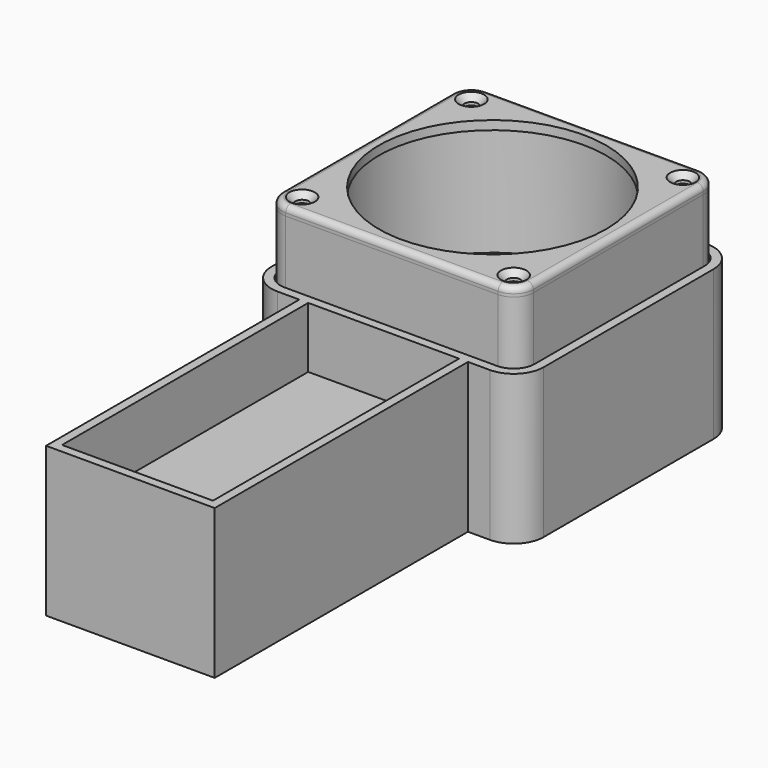
from build123d import *

# Parameters (mm, degrees)
F0_W      = 80
F0_H      = 80
F0_R      = 2.1
F0_R_2    = 38.4
F1_DEPTH  = 25
F2_W      = 79.6
F2_H      = 79.6
F2_R      = 2.3
F2_R_2    = 38.6
F3_DEPTH  = 1.5875
F4_W      = 79.6
F4_H      = 79.6
F4_R      = 2.3
F4_R_2    = 38.6
F5_DEPTH  = 1.5875
F8_W      = 92
F8_H      = 92
F8_W_2    = 86
F8_H_2    = 86
F9_DEPTH  = 27.54
F10_W     = 92
F10_H     = 92
F10_R     = 2.3
F10_R_2   = 38.4
F11_DEPTH = 3
F12_SIZE  = 2
F13_W     = 92
F13_H     = 92
F13_W_2   = 86
F13_H_2   = 86
F14_DEPTH = 20
F15_R     = 42.4
F15_R_2   = 38.4
F16_DEPTH = 1.27
F17_R     = 42.2
F17_R_2   = 38.6
F18_DEPTH = 1.5875
F19_W     = 85
F19_H     = 85
F19_R     = 38.4
F20_DEPTH = 41
F21_R     = 41.4
F22_DEPTH = 38
F23_R     = 3.25
F24_DEPTH = 12.7
F25_R     = 3.15
F26_DEPTH = 6.7
F27_R     = 3.6661742094
F28_DEPTH = 0.5
F30_DEPTH = 71.8585
F31_R     = 6.6
F32_R     = 2
F33_R     = 2.3
F33_R_2   = 38.4
F34_DEPTH = 3
F35_SIZE  = 2
F36_R     = 2
F37_R     = 7.1
F38_R     = 10.1
F39_R     = 7.1
F40_W     = 57
F40_H     = 107
F41_DEPTH = 30
F42_W     = 51
F42_H     = 104
F43_DEPTH = 27
F44_W     = 57
F44_H     = 110
F44_W_2   = 51
F44_H_2   = 104
F45_DEPTH = 20.54


with BuildPart() as f1:
    # F0 (on Top) → F1 (new body)
    with BuildSketch(Plane.XY):
        Rectangle(F0_W, F0_H)
        with Locations((-35.75, -35.75)):
            Circle(F0_R, mode=Mode.SUBTRACT)
        with Locations((35.75, -35.75)):
            Circle(F0_R, mode=Mode.SUBTRACT)
        with Locations((-35.75, 35.75)):
            Circle(F0_R, mode=Mode.SUBTRACT)
        Circle(F0_R_2, mode=Mode.SUBTRACT)
        with Locations((35.75, 35.75)):
            Circle(F0_R, mode=Mode.SUBTRACT)
    extrude(amount=F1_DEPTH)


with BuildPart() as f3:
    # F2 (on face) → F3 (new body)
    with BuildSketch(Plane.XY.offset(25)):
        Rectangle(F2_W, F2_H)
        with Locations((-35.75, -35.75)):
            Circle(F2_R, mode=Mode.SUBTRACT)
        with Locations((35.75, -35.75)):
            Circle(F2_R, mode=Mode.SUBTRACT)
        with Locations((-35.75, 35.75)):
            Circle(F2_R, mode=Mode.SUBTRACT)
        Circle(F2_R_2, mode=Mode.SUBTRACT)
        with Locations((35.75, 35.75)):
            Circle(F2_R, mode=Mode.SUBTRACT)
    extrude(amount=F3_DEPTH)


with BuildPart() as f5:
    # F4 (on face) → F5 (new body)
    with BuildSketch(Plane(origin=(0, 0, 0), x_dir=(1, 0, 0), z_dir=(0, 0, -1))):
        Rectangle(F4_W, F4_H)
        with Locations((-35.75, -35.75)):
            Circle(F4_R, mode=Mode.SUBTRACT)
        with Locations((35.75, -35.75)):
            Circle(F4_R, mode=Mode.SUBTRACT)
        with Locations((-35.75, 35.75)):
            Circle(F4_R, mode=Mode.SUBTRACT)
        Circle(F4_R_2, mode=Mode.SUBTRACT)
        with Locations((35.75, 35.75)):
            Circle(F4_R, mode=Mode.SUBTRACT)
    extrude(amount=F5_DEPTH)


with BuildPart() as f9:
    # F8 (on offset) → F9 (new body, through all)
    with BuildSketch(Plane.XY.offset(26.27)):
        Rectangle(F8_W, F8_H)
        Rectangle(F8_W_2, F8_H_2, mode=Mode.SUBTRACT)
    extrude(amount=-F9_DEPTH)

    # F10 (on face) → F11 (join)
    with BuildSketch(Plane.XY.offset(26.27)):
        Rectangle(F10_W, F10_H)
        with Locations((-35.75, -35.75)):
            Circle(F10_R, mode=Mode.SUBTRACT)
        with Locations((35.75, -35.75)):
            Circle(F10_R, mode=Mode.SUBTRACT)
        with Locations((-35.75, 35.75)):
            Circle(F10_R, mode=Mode.SUBTRACT)
        Circle(F10_R_2, mode=Mode.SUBTRACT)
        with Locations((35.75, 35.75)):
            Circle(F10_R, mode=Mode.SUBTRACT)
    extrude(amount=F11_DEPTH)

    # F12
    f12_edges = [f9.edges().sort_by_distance(p)[0] for p in [
        (33.45, 35.75, 29.27),
        (33.45, -35.75, 29.27),
        (-38.05, -35.75, 29.27),
        (-38.05, 35.75, 29.27),
    ]]
    chamfer(f12_edges, length=F12_SIZE)

    # F13 (on face) → F14 (join)
    with BuildSketch(Plane.XY.offset(29.27)):
        Rectangle(F13_W, F13_H)
        Rectangle(F13_W_2, F13_H_2, mode=Mode.SUBTRACT)
    extrude(amount=F14_DEPTH)

    # F15 (on face) → F16 (cut)
    with BuildSketch(Plane.XY.offset(29.27)):
        Circle(F15_R)
        Circle(F15_R_2, mode=Mode.SUBTRACT)
    extrude(amount=-F16_DEPTH, mode=Mode.SUBTRACT)

    # F37
    f37_edges = [f9.edges().sort_by_distance(p)[0] for p in [
        (-43, -43, 39.27),
        (-43, 43, 39.27),
        (43, 43, 39.27),
        (43, -43, 39.27),
    ]]
    fillet(f37_edges, radius=F37_R)

    # F38
    f38_edges = [f9.edges().sort_by_distance(p)[0] for p in [
        (46, -46, 24),
        (46, 46, 24),
        (-46, 46, 24),
        (-46, -46, 24),
    ]]
    fillet(f38_edges, radius=F38_R)

    # F39
    f39_edges = [f9.edges().sort_by_distance(p)[0] for p in [
        (-43, -43, 12.5),
        (43, -43, 12.5),
        (-43, 43, 12.5),
        (43, 43, 12.5),
    ]]
    fillet(f39_edges, radius=F39_R)

    # F40 (on face) → F41 (join)
    with BuildSketch(Plane(origin=(0, 0, -1.27), x_dir=(1, 0, 0), z_dir=(0, 0, -1))):
        with Locations((0, 99.5)):
            Rectangle(F40_W, F40_H)
    extrude(amount=-F41_DEPTH)

    # F42 (on face) → F43 (cut)
    with BuildSketch(Plane(origin=(0, 0, -1.27), x_dir=(1, 0, 0), z_dir=(0, 0, -1))):
        with Locations((0, 98)):
            Rectangle(F42_W, F42_H)
    extrude(amount=-F43_DEPTH, mode=Mode.SUBTRACT)

    # F44 (on face) → F45 (join, through all)
    with BuildSketch(Plane.XY.offset(28.73)):
        with Locations((0, -98)):
            Rectangle(F44_W, F44_H)
        with Locations((0, -98)):
            Rectangle(F44_W_2, F44_H_2, mode=Mode.SUBTRACT)
    extrude(amount=F45_DEPTH)


with BuildPart() as f18:
    # F17 (on face) → F18 (new body)
    with BuildSketch(Plane.XY.offset(28)):
        Circle(F17_R)
        Circle(F17_R_2, mode=Mode.SUBTRACT)
    extrude(amount=F18_DEPTH)


with BuildPart() as f20:
    # F19 (on face) → F20 (new body)
    with BuildSketch(Plane.XY.offset(29.27)):
        Rectangle(F19_W, F19_H)
        Circle(F19_R, mode=Mode.SUBTRACT)
    extrude(amount=F20_DEPTH)

    # F21 (on face) → F22 (cut)
    with BuildSketch(Plane.XY.offset(70.27)):
        Circle(F21_R)
    extrude(amount=-F22_DEPTH, mode=Mode.SUBTRACT)

    # F23 (on face) → F24 (cut)
    with BuildSketch(Plane(origin=(0, 0, 29.27), x_dir=(1, 0, 0), z_dir=(0, 0, -1))):
        with Locations((35.75, -35.75)):
            Circle(F23_R)
        with Locations((-35.75, 35.75)):
            Circle(F23_R)
        with Locations((-35.75, -35.75)):
            Circle(F23_R)
        with Locations((35.75, 35.75)):
            Circle(F23_R)
    extrude(amount=-F24_DEPTH, mode=Mode.SUBTRACT)

    # F25 (on face) → F26 (cut)
    with BuildSketch(Plane.XY.offset(70.27)):
        with Locations((-35.75, 35.75)):
            Circle(F25_R)
        with Locations((35.75, 35.75)):
            Circle(F25_R)
        with Locations((35.75, -35.75)):
            Circle(F25_R)
        with Locations((-35.75, -35.75)):
            Circle(F25_R)
    extrude(amount=-F26_DEPTH, mode=Mode.SUBTRACT)

    # F27 (on face) → F28 (cut)
    with BuildSketch(Plane.XY.offset(70.27)):
        with Locations((-35.75, 35.75)):
            Circle(F27_R)
        with Locations((-35.75, -35.75)):
            Circle(F27_R)
        with Locations((35.75, -35.75)):
            Circle(F27_R)
        with Locations((35.75, 35.75)):
            Circle(F27_R)
    extrude(amount=-F28_DEPTH, mode=Mode.SUBTRACT)

    # F29 (on face) → F30 (cut, through all)
    with BuildSketch(Plane.XY.offset(70.27)):
        with BuildLine():
            ThreePointArc((-33.040767305, 29.659192435), (-36.3455933225, 29.1104859226), (-39.5, 30.2386137325))
            Line((-39.5, 30.2386137325), (-39.5, 20.2758477011))
            ThreePointArc((-39.5, 20.2758477011), (-36.572565126, 25.1755333628), (-33.040767305, 29.659192435))
        make_face()
        with BuildLine():
            ThreePointArc((-33.040767305, -29.659192435), (-36.572565126, -25.1755333628), (-39.5, -20.2758477011))
            Line((-39.5, -20.2758477011), (-39.5, -30.2386137325))
            ThreePointArc((-39.5, -30.2386137325), (-36.3455933225, -29.1104859226), (-33.040767305, -29.659192435))
        make_face()
        with BuildLine():
            ThreePointArc((-30.2386137325, 39.5), (-29.1104859226, 36.3455933225), (-29.659192435, 33.040767305))
            ThreePointArc((-29.659192435, 33.040767305), (-25.1755333628, 36.572565126), (-20.2758477011, 39.5))
            Line((-20.2758477011, 39.5), (-30.2386137325, 39.5))
        make_face()
        with BuildLine():
            ThreePointArc((-29.659192435, -33.040767305), (-29.1104859226, -36.3455933225), (-30.2386137325, -39.5))
            Line((-30.2386137325, -39.5), (-20.2758477011, -39.5))
            ThreePointArc((-20.2758477011, -39.5), (-25.1755333628, -36.572565126), (-29.659192435, -33.040767305))
        make_face()
        with BuildLine():
            ThreePointArc((29.659192435, -33.040767305), (25.1755333628, -36.572565126), (20.2758477011, -39.5))
            Line((20.2758477011, -39.5), (30.2386137325, -39.5))
            ThreePointArc((30.2386137325, -39.5), (29.1104859226, -36.3455933225), (29.659192435, -33.040767305))
        make_face()
        with BuildLine():
            ThreePointArc((33.040767305, -29.659192435), (36.3455933225, -29.1104859226), (39.5, -30.2386137325))
            Line((39.5, -30.2386137325), (39.5, -20.2758477011))
            ThreePointArc((39.5, -20.2758477011), (36.572565126, -25.1755333628), (33.040767305, -29.659192435))
        make_face()
        with BuildLine():
            ThreePointArc((33.040767305, 29.659192435), (36.572565126, 25.1755333628), (39.5, 20.2758477011))
            Line((39.5, 20.2758477011), (39.5, 30.2386137325))
            ThreePointArc((39.5, 30.2386137325), (36.3455933225, 29.1104859226), (33.040767305, 29.659192435))
        make_face()
        with BuildLine():
            ThreePointArc((29.659192435, 33.040767305), (29.1104859226, 36.3455933225), (30.2386137325, 39.5))
            Line((30.2386137325, 39.5), (20.2758477011, 39.5))
            ThreePointArc((20.2758477011, 39.5), (25.1755333628, 36.572565126), (29.659192435, 33.040767305))
        make_face()
    extrude(amount=-F30_DEPTH, mode=Mode.SUBTRACT)

    # F31
    f31_edges = [f20.edges().sort_by_distance(p)[0] for p in [
        (42.5, -42.5, 49.77),
        (-42.5, -42.5, 49.77),
        (42.5, 42.5, 49.77),
        (-42.5, 42.5, 49.77),
    ]]
    fillet(f31_edges, radius=F31_R)

    # F32
    f32_edges = [f20.edges().sort_by_distance(p)[0] for p in [
        (0, 42.5, 29.27),
    ]]
    fillet(f32_edges, radius=F32_R)


with BuildPart() as f34:
    # F33 (on face) → F34 (new body)
    with BuildSketch(Plane.XY.offset(70.27)):
        with BuildLine():
            ThreePointArc((35.9, -42.5), (40.5669047558, -40.5669047558), (42.5, -35.9))
            Line((42.5, -35.9), (42.5, 35.9))
            ThreePointArc((42.5, 35.9), (40.5669047558, 40.5669047558), (35.9, 42.5))
            Line((35.9, 42.5), (-35.9, 42.5))
            ThreePointArc((-35.9, 42.5), (-40.5669047558, 40.5669047558), (-42.5, 35.9))
            Line((-42.5, 35.9), (-42.5, -35.9))
            ThreePointArc((-42.5, -35.9), (-40.5669047558, -40.5669047558), (-35.9, -42.5))
            Line((-35.9, -42.5), (35.9, -42.5))
        make_face()
        with Locations((-35.75, -35.75)):
            Circle(F33_R, mode=Mode.SUBTRACT)
        with Locations((35.75, -35.75)):
            Circle(F33_R, mode=Mode.SUBTRACT)
        with Locations((-35.75, 35.75)):
            Circle(F33_R, mode=Mode.SUBTRACT)
        Circle(F33_R_2, mode=Mode.SUBTRACT)
        with Locations((35.75, 35.75)):
            Circle(F33_R, mode=Mode.SUBTRACT)
    extrude(amount=F34_DEPTH)

    # F35
    f35_edges = [f34.edges().sort_by_distance(p)[0] for p in [
        (33.45, 35.75, 73.27),
        (-38.05, 35.75, 73.27),
        (-38.05, -35.75, 73.27),
        (33.45, -35.75, 73.27),
    ]]
    chamfer(f35_edges, length=F35_SIZE)

    # F36
    f36_edges = [f34.edges().sort_by_distance(p)[0] for p in [
        (42.5, 0, 73.27),
        (40.566905, -40.566905, 73.27),
        (40.566905, 40.566905, 73.27),
        (0, 42.5, 73.27),
        (-40.566905, 40.566905, 73.27),
        (-42.5, 0, 73.27),
        (-40.566905, -40.566905, 73.27),
        (0, -42.5, 73.27),
    ]]
    fillet(f36_edges, radius=F36_R)


solid = Compound([f1.part, f3.part, f5.part, f9.part, f18.part, f20.part, f34.part])
